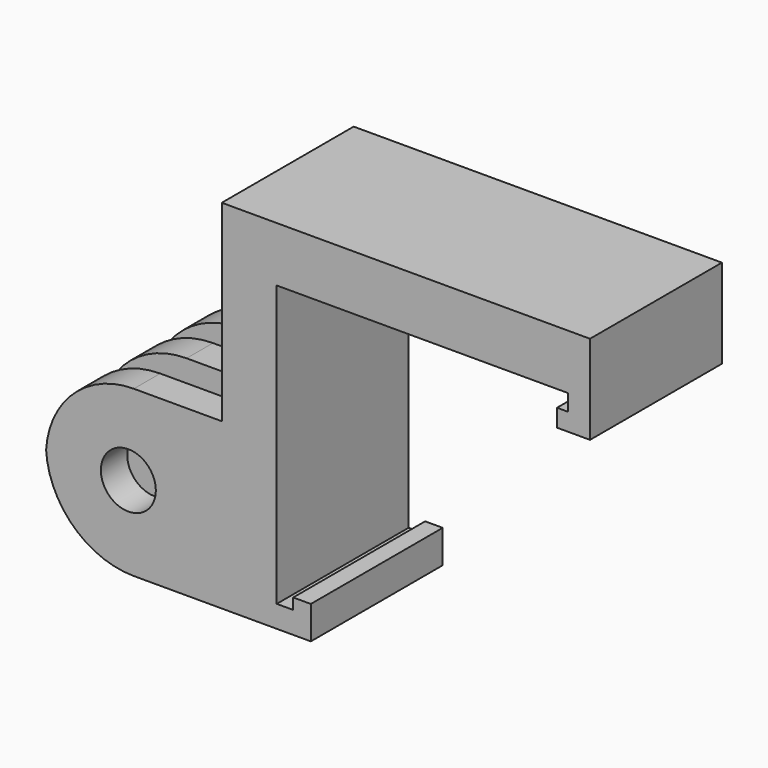
from build123d import *

# Parameters (mm, degrees)
F1_DEPTH    = 15
F2_W        = 3
F2_H        = 15
F3_DEPTH    = 16
F5_DEPTH    = 25
F6_T1_DEPTH = 43
F6_T3_DEPTH = 43
F6_T5_DEPTH = 43


# Not quite as in the source:
# - a fillet or chamfer that OpenCascade refuses, or shapes differently, is made with other operations: its cross-section is extruded or revolved along the edge and cut away or added


with BuildPart() as f1:
    # F0 (on Front) → F1 (new body)
    with BuildSketch(Plane.XZ):
        Polygon((0, -23.585311383), (0, 0), (25, 0), (26.5, 0), (26.5, -1.5), (25.5, -1.5), (25.5, -3.1), (28.5, -3.1), (28.5, 5), (25, 5), (-5, 5), (-5, -24), (-5, -25.5), (-5, -27.5), (0, -27.5), (3.1, -27.5), (3.1, -24.5), (1.5, -24.5), (1.5, -25.5), (0, -25.5), (0, -25.085311383), align=None)
    extrude(amount=F1_DEPTH)

    # F2 (on face) → F3 (join)
    with BuildSketch(Plane(origin=(-5, 0, 0), x_dir=(0, -1, 0), z_dir=(-1, 0, 0))):
        with Locations((1.5, -20)):
            Rectangle(F2_W, F2_H)
        with Locations((7.5, -20)):
            Rectangle(F2_W, F2_H)
        with Locations((13.5, -20)):
            Rectangle(F2_W, F2_H)
    extrude(amount=F3_DEPTH)

    # F4 (on face) → F5 (cut)
    with BuildSketch(Plane.XZ.offset(15)):
        with BuildLine():
            ThreePointArc((-16, -20), (-13.5, -22.5), (-11, -20))
            ThreePointArc((-11, -20), (-13.5, -17.5), (-16, -20))
        make_face()
    extrude(amount=-F5_DEPTH, mode=Mode.SUBTRACT)

    # F6: fillet of radius 8 on 5 edges, made by hand

    # F6_s2 → F6_t1 (cut)
    with BuildSketch(Plane.XZ.offset(-8)):
        with BuildLine():
            ThreePointArc((-21, -20.5), (-18.6568542495, -14.8431457505), (-13, -12.5))
            Line((-13, -12.5), (-21, -12.5))
            Line((-21, -12.5), (-21, -20.5))
        make_face()
    extrude(amount=F6_T1_DEPTH, mode=Mode.SUBTRACT)

    # F6_s4 → F6_t3 (cut)
    with BuildSketch(Plane.XZ.offset(-14)):
        with BuildLine():
            ThreePointArc((-21, -20.5), (-18.6568542495, -14.8431457505), (-13, -12.5))
            Line((-13, -12.5), (-21, -12.5))
            Line((-21, -12.5), (-21, -20.5))
        make_face()
        with BuildLine():
            ThreePointArc((-13, -27.5), (-18.6568542495, -25.1568542495), (-21, -19.5))
            Line((-21, -19.5), (-21, -27.5))
            Line((-21, -27.5), (-13, -27.5))
        make_face()
    extrude(amount=F6_T3_DEPTH, mode=Mode.SUBTRACT)

    # F6_s6 → F6_t5 (cut)
    with BuildSketch(Plane.XZ.offset(-20)):
        with BuildLine():
            ThreePointArc((-21, -20.5), (-18.6568542495, -14.8431457505), (-13, -12.5))
            Line((-13, -12.5), (-21, -12.5))
            Line((-21, -12.5), (-21, -20.5))
        make_face()
        with BuildLine():
            ThreePointArc((-13, -27.5), (-18.6568542495, -25.1568542495), (-21, -19.5))
            Line((-21, -19.5), (-21, -27.5))
            Line((-21, -27.5), (-13, -27.5))
        make_face()
    extrude(amount=F6_T5_DEPTH, mode=Mode.SUBTRACT)


solid = f1.part
